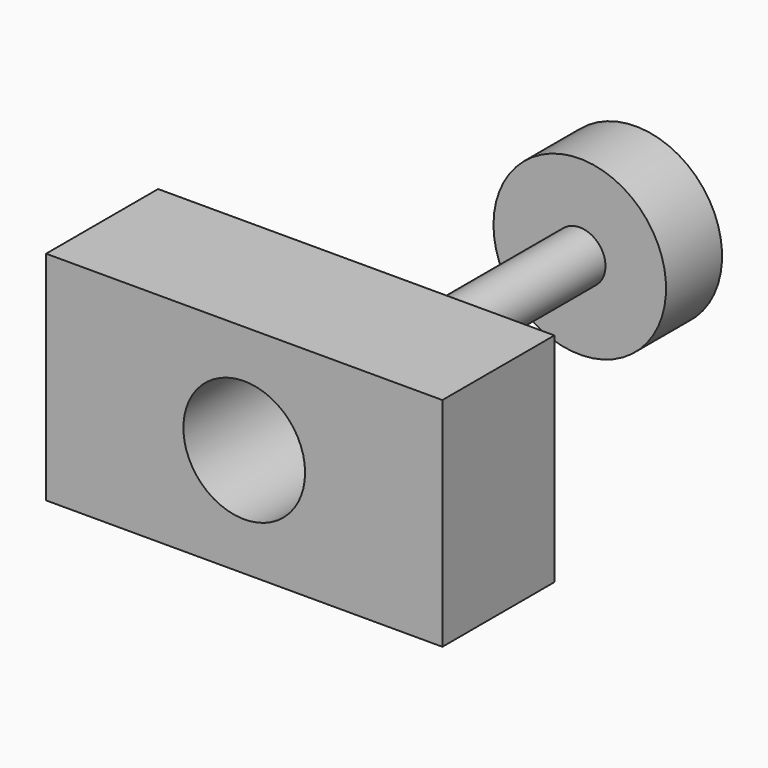
from build123d import *

# Parameters (mm, degrees)
F0_W     = 71.8886852264
F0_H     = 39.4034199417
F0_R     = 11.0373751876
F1_DEPTH = 25.4
F2_W     = 4.6622366644
F2_H     = 30.9813190252
F4_R     = 15.6540628249
F5_DEPTH = 12.7


with BuildPart() as f1:
    # F0 (on Front) → F1 (new body)
    with BuildSketch(Plane.XZ):
        Rectangle(F0_W, F0_H)
        Circle(F0_R, mode=Mode.SUBTRACT)
    extrude(amount=F1_DEPTH)


with BuildPart() as f3:
    # F2 (on Top) → F3 (revolve)
    with BuildSketch(Plane.XY):
        with Locations((-2.3311183322, 35.1923694834)):
            Rectangle(F2_W, F2_H)
    revolve(axis=Axis((0, 35.1923694834, 0), (0, -1, 0)))

    # F4 (on face) → F5 (join)
    with BuildSketch(Plane(origin=(0, 50.683028996, 0), x_dir=(-1, 0, 0), z_dir=(0, 1, 0))):
        Circle(F4_R)
    extrude(amount=F5_DEPTH)


solid = Compound([f1.part, f3.part])
